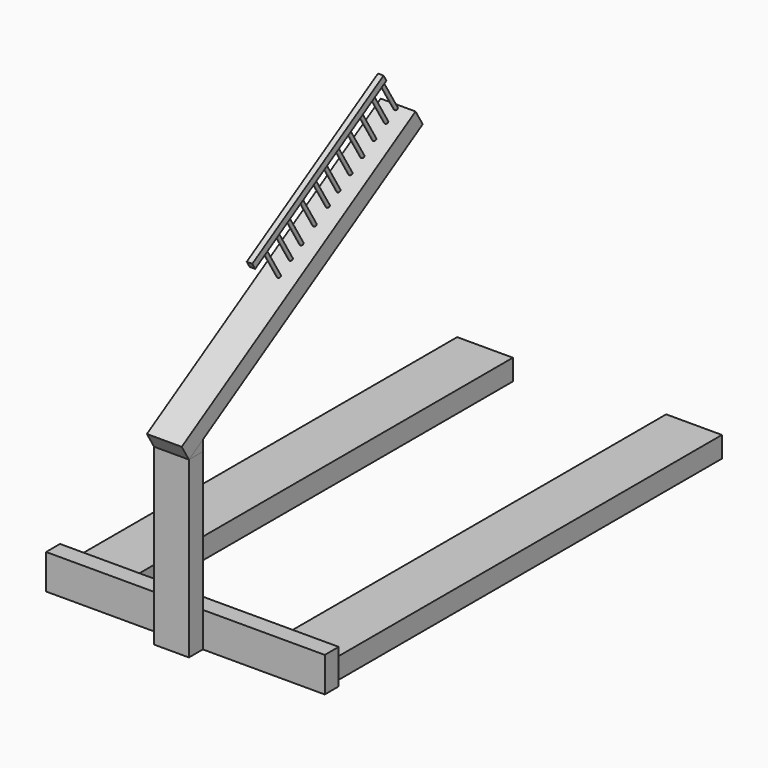
from build123d import *

# Parameters (mm, degrees)
F0_W      = 40.64
F0_H      = 355.6
F2_DEPTH  = 15.24
F1_W      = 203.2
F1_H      = 25.4
F3_DEPTH  = 12.7
F4_W      = 25.4
F4_H      = 25.4
F4_H_2    = 101.6
F5_DEPTH  = 12.7
F7_DEPTH  = 25.4
F9_DEPTH  = 25.4
F10_R     = 1.27
F11_DEPTH = 25.4
F12_W     = 4.064
F12_H     = 139.7
F13_DEPTH = 5.08


with BuildPart() as f2:
    # F0 (on Top) → F2 (new body)
    with BuildSketch(Plane.XY):
        with Locations((177.8, 177.8)):
            Rectangle(F0_W, F0_H)
    extrude(amount=F2_DEPTH)


with BuildPart() as f2b:
    # F0 (on Top) → F2, piece 2 (new body)
    with BuildSketch(Plane.XY):
        with Locations((25.4, 177.8)):
            Rectangle(F0_W, F0_H)
    extrude(amount=F2_DEPTH)


with BuildPart() as f3:
    # F1 (on Front) → F3 (new body)
    with BuildSketch(Plane.XZ):
        with Locations((101.6, 12.7)):
            Rectangle(F1_W, F1_H)
    extrude(amount=F3_DEPTH)

    # F4 (on face) → F5 (join)
    with BuildSketch(Plane.XZ.offset(12.7)):
        with Locations((101.6, 12.7)):
            Rectangle(F4_W, F4_H)
        with Locations((101.6, 76.2)):
            Rectangle(F4_W, F4_H_2)
    extrude(amount=F5_DEPTH)


with BuildPart() as f7:
    # F6 (on face) → F7 (new body)
    with BuildSketch(Plane.YZ.offset(114.3)):
        Polygon((181.1396062945, 266.5128934246), (-31.9632804674, 137.8725962634), (-25.4, 127), (-12.7, 134.666399075), (187.7028867619, 255.6402971612), align=None)
    extrude(amount=-F7_DEPTH)

    # F10 (on face) → F11 (join)
    with BuildSketch(Plane(origin=(0, -69.5359015573, 115.1917531478), x_dir=(1, 0, 0), z_dir=(0, -0.5167937376, 0.856109942))):
        with Locations((101.6, 290.2676121474)):
            Circle(F10_R)
        with Locations((101.6, 267.4076121474)):
            Circle(F10_R)
        with Locations((101.6, 242.0076121474)):
            Circle(F10_R)
        with Locations((101.6, 217.8776121474)):
            Circle(F10_R)
        with Locations((101.6, 203.9076121474)):
            Circle(F10_R)
        with Locations((101.6, 189.9376121474)):
            Circle(F10_R)
        with Locations((101.6, 178.5076121474)):
            Circle(F10_R)
        with Locations((101.6, 165.8076121474)):
            Circle(F10_R)
        with Locations((101.6, 229.3076121474)):
            Circle(F10_R)
        with Locations((101.6, 254.7076121474)):
            Circle(F10_R)
        with Locations((101.6, 280.1076121474)):
            Circle(F10_R)
    extrude(amount=F11_DEPTH)

    # F12 (on face) → F13 (join)
    with BuildSketch(Plane(origin=(0, -82.6624624921, 136.9369456745), x_dir=(1, 0, 0), z_dir=(0, -0.5167937376, 0.856109942))):
        with Locations((101.6330005474, 222.8175677299)):
            Rectangle(F12_W, F12_H)
    extrude(amount=F13_DEPTH)


with BuildPart() as f9:
    # F8 (on face) → F9 (new body)
    with BuildSketch(Plane.YZ.offset(114.3)):
        Polygon((-25.4, 127), (-12.7, 127), (-12.7, 134.666399075), align=None)
    extrude(amount=-F9_DEPTH)


solid = Compound([f2.part, f2b.part, f3.part, f7.part, f9.part])
